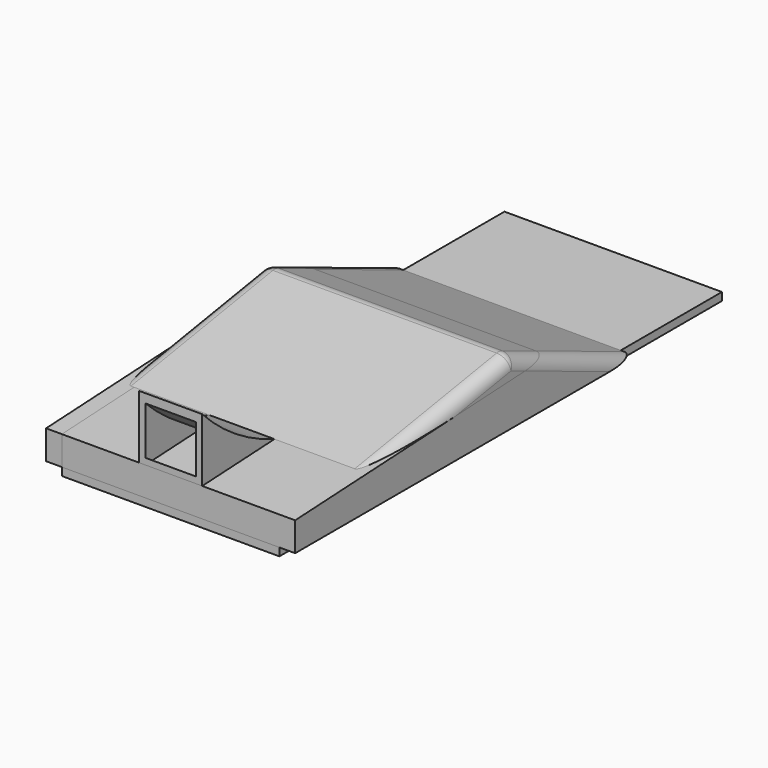
from build123d import *

# Parameters (mm, degrees)
F0_W      = 87.376
F0_H      = 222.25
F1_DEPTH  = 3.175
F3_DEPTH  = 6.35
F4_DEPTH  = 87.376
F5_DEPTH  = 6.35
F7_DEPTH  = 100.076
F8_W      = 37.338
F8_H      = 25.4
F9_DEPTH  = 38.1
F10_W     = 82.1538120508
F10_H     = 215.1187956333
F11_DEPTH = 0.0254
F13_DEPTH = 38.1
F14_T     = -2.54
F15_DEPTH = 25.4
F16_R     = 5.08
F16_2_R   = 5.08
F16_3_R   = 5.08


# Not quite as in the source:
# - a feature names something its author has since deleted; it is built from what else it names


with BuildPart() as f1:
    # F0 (on Top) → F1 (new body)
    with BuildSketch(Plane.XY):
        Rectangle(F0_W, F0_H)
    extrude(amount=F1_DEPTH)

    # F10 (on face) → F11 (cut)
    with BuildSketch(Plane(origin=(0, 0, 0), x_dir=(1, 0, 0), z_dir=(0, 0, -1))):
        Rectangle(F10_W, F10_H)
    extrude(amount=-F11_DEPTH, mode=Mode.SUBTRACT)


with BuildPart() as f3:
    # F2 (on face) → F3 (new body)
    with BuildSketch(Plane(origin=(-43.688, 0, 0), x_dir=(0, -1, 0), z_dir=(-1, 0, 0))):
        Polygon((-16.2016954273, 21.3054399937), (-60.325, 3.175), (111.125, 3.175), (111.125, 14.8184783757), align=None)
    extrude(amount=F3_DEPTH)


with BuildPart() as f4:
    # F4 (new): a face of the model
    f4_faces = [f3.part.faces().sort_by_distance(p)[0] for p in [
        (-43.688, -29.9876869661, 10.4717867794),
    ]]
    extrude(f4_faces, amount=F4_DEPTH)

    # F5 (add): a face of the model
    f5_faces = [f4.faces().sort_by_distance(p)[0] for p in [
        (43.688, -29.9876869661, 10.4717867794),
    ]]
    extrude(f5_faces, amount=F5_DEPTH)


with BuildPart() as f7:
    # F6 (on face) → F7 (new body)
    with BuildSketch(Plane.YZ.offset(50.038)):
        with BuildLine():
            Line((-111.125, 40.2184783757), (-111.125, 14.8184783757))
            Line((-111.125, 14.8184783757), (-74.8663830833, 16.6657599334))
            ThreePointArc((-74.8663830833, 16.6657599334), (-94.3214065955, 26.4012254718), (-111.125, 40.2184783757))
        make_face()
    extrude(amount=-F7_DEPTH)

    # F8 (on face) → F9 (cut)
    with BuildSketch(Plane.XZ.offset(111.125)):
        Polygon((-50.038, 14.8184783757), (-50.038, 40.2184783757), (-12.7, 40.2184783757), (-12.7, 47.7892234921), (-50.038, 45.227330178), (-81.4004353094, 16.6523270309), align=None)
        with Locations((-31.369, 27.5184783757)):
            Rectangle(F8_W, F8_H)
        Polygon((12.7, 47.7892234921), (12.7, 40.2184783757), (50.038, 40.2184783757), (50.038, 14.8184783757), (75.860601027, 14.8184783757), (72.0834517309, 16.6523270309), (65.1312917471, 48.7745702267), (40.7210164215, 45.227330178), align=None)
        Polygon((50.038, 40.2184783757), (12.7, 40.2184783757), (12.7, 14.8184783757), (46.51265473, 14.8184783757), (50.038, 14.8184783757), align=None)
    extrude(amount=-F9_DEPTH, mode=Mode.SUBTRACT)

    # F14
    f14_openings = [f7.faces().sort_by_distance(p)[0] for p in [
        (0, -111.125, 27.518478),
    ]]
    offset(amount=F14_T, openings=f14_openings)

    # F15 (cut): a face of the model
    f15_faces = [f7.faces().sort_by_distance(p)[0] for p in [
        (0, -98.4966020741, 18.0051564926),
    ]]
    extrude(f15_faces, amount=-F15_DEPTH, mode=Mode.SUBTRACT)


with BuildPart() as f7b:
    # F6 (on face) → F7, piece 2 (new body)
    with BuildSketch(Plane.YZ.offset(50.038)):
        Polygon((-2.1756697122, 28.8567718609), (-74.8663830833, 16.6657599334), (16.2016954273, 21.3054399937), align=None)
    extrude(amount=-F7_DEPTH)


with BuildPart() as f13_tool:
    # F12 (on Right) → F13 (new body, symmetric)
    with BuildSketch(Plane.YZ):
        Polygon((-105.6373342872, 0), (54.759632796, 0), (-3.2019854989, 24.5833210647), (-77.8798013926, 12.2278658673), (-105.6373342872, 12.2278658673), align=None)
    extrude(amount=F13_DEPTH, both=True)


with BuildPart() as f1_1:
    add(f1.part)

    # F13: cut by f13_tool
    add(f13_tool.part, mode=Mode.SUBTRACT)


with BuildPart() as f4_1:
    add(f4.part)

    # F13: cut by f13_tool
    add(f13_tool.part, mode=Mode.SUBTRACT)

    # F16#2
    f16_2_edges = [f4_1.edges().sort_by_distance(p)[0] for p in [
        (50.038, 38.263348, 12.24022),
    ]]
    fillet(f16_2_edges, radius=F16_2_R)


with BuildPart() as f7b_1:
    add(f7b.part)

    # F13: cut by f13_tool
    add(f13_tool.part, mode=Mode.SUBTRACT)

    # F16#3
    f16_3_edges = [f7b_1.edges().sort_by_distance(p)[0] for p in [
        (-50.038, 7.013013, 25.081106),
        (-50.038, -38.521026, 22.761266),
        (50.038, 7.013013, 25.081106),
        (50.038, -38.521026, 22.761266),
        (0, -2.17567, 28.856772),
    ]]
    fillet(f16_3_edges, radius=F16_3_R)


with BuildPart() as f3_1:
    add(f3.part)

    # F16
    f16_edges = [f3_1.edges().sort_by_distance(p)[0] for p in [
        (-50.038, 38.263348, 12.24022),
    ]]
    fillet(f16_edges, radius=F16_R)


solid = Compound([f7.part, f1_1.part, f4_1.part, f7b_1.part, f3_1.part])
